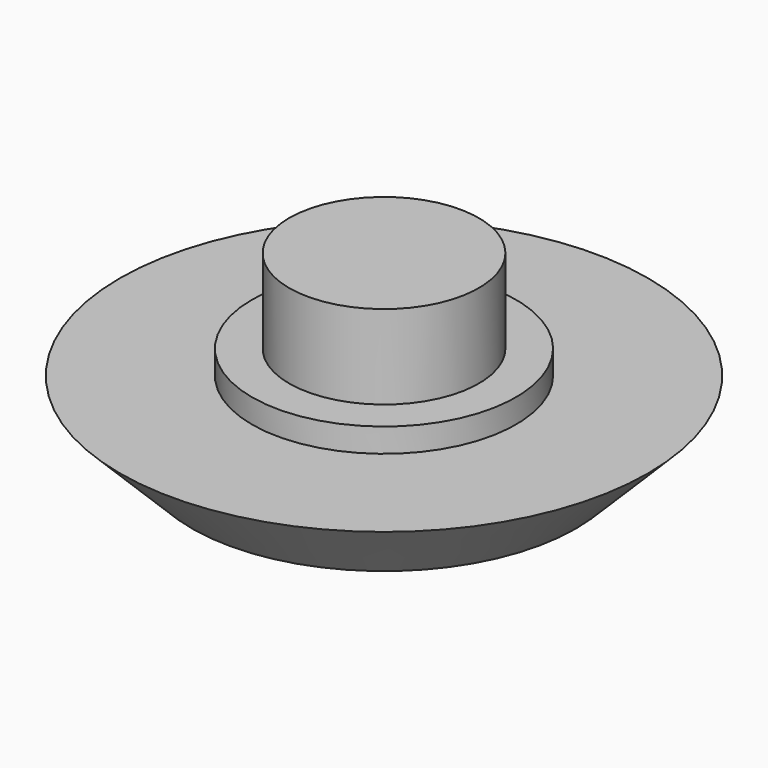
from build123d import *

# Parameters (mm, degrees)
F2_SIZE      = 2.99999
F3_TEXT_SIZE = 8.3130907216
F4_TEXT_SIZE = 7.5662114088
F5_DEPTH     = 0.1


# Not quite as in the source:
# - a fillet or chamfer is up to 0.001 mm smaller than in the source, because OpenCascade refuses the exact size
# - Text() gives the source's letters only with a copy of the font that has no kerning and outlines rounded to 1/6400 em; it was checked with that copy


with BuildPart() as f1:
    # F0 (on Front) → F1 (revolve)
    with BuildSketch(Plane.XZ):
        Polygon((0, 0), (0, 7.5), (-3.95, 7.5), (-3.95, 4), (-5.5, 4), (-5.5, 3), (-11, 3), (-11, 0), align=None)
    revolve(axis=Axis((0, 0, 3.75), (0, 0, 1)))

    # F2 (size 3 in the source; OpenCascade refuses exactly that, so slightly less here)
    f2_edges = [f1.edges().sort_by_distance(p)[0] for p in [
        (11, 0, 0),
    ]]
    chamfer(f2_edges, length=F2_SIZE)

    # F3 (on face) + F4 (on face) → F5 (cut)
    with BuildSketch(Plane(origin=(0, 0, 0), x_dir=(1, 0, 0), z_dir=(0, 0, -1))):
        with Locations((-8.0546053359, -3.0979251314)):
            Text('R', F3_TEXT_SIZE, font='Open Sans', text_align=(TextAlign.LEFT, TextAlign.BOTTOM))
    with BuildSketch(Plane(origin=(0, 0, 0), x_dir=(1, 0, 0), z_dir=(0, 0, -1))):
        with Locations((2.9810222331, -2.9108805757)):
            Text('C', F4_TEXT_SIZE, font='Open Sans', text_align=(TextAlign.LEFT, TextAlign.BOTTOM))
    extrude(amount=-F5_DEPTH, mode=Mode.SUBTRACT)


solid = f1.part
